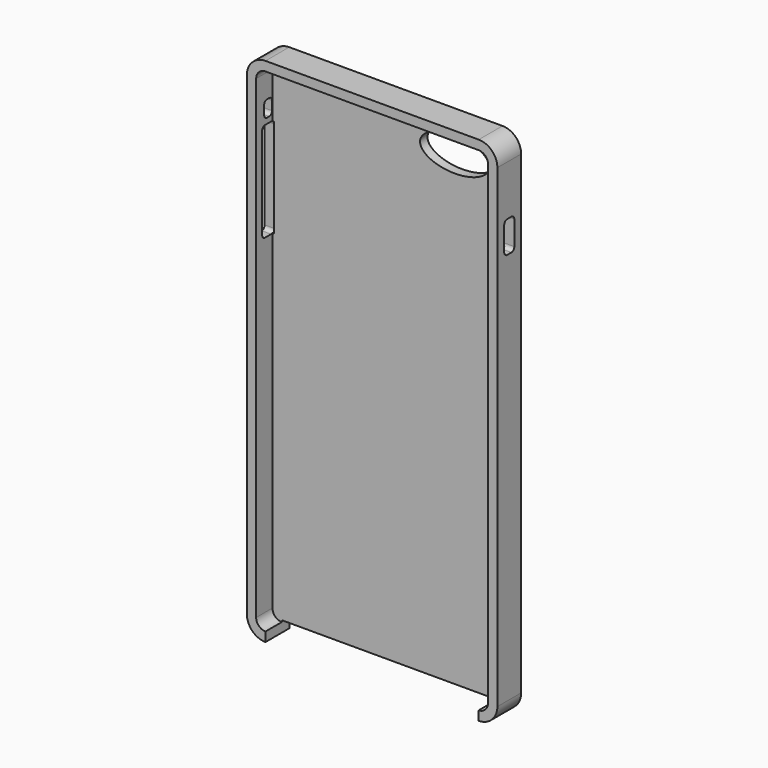
from build123d import *

# Parameters (mm, degrees)
F0_W          = 68.3
F0_H          = 139.5
F1_DEPTH      = 4.05
F2_R          = 5.08
F3_T          = -2.54
F5_DEPTH      = 30
F7_W          = 32.1311485022
F7_H          = 8.1
F8_DEPTH      = 3
F9_W          = 3.4326917958
F9_H          = 8.6012896579
F10_DEPTH     = 3
F11_W         = 2.6687926147
F11_H         = 4.4363630507
F12_DEPTH     = 3
F13_W         = 4.0359543636
F13_H         = 27.0408764482
F14_DEPTH     = 3
F15_W         = 16.4470494014
F15_H         = 8.1
F8_FACE_W     = 9.5618020964
F8_FACE_H     = 8.1
F16_DEPTH     = 3
F19_T1_DEPTH  = 2.54
F19_T3_DEPTH  = 2.54
F19_T8_DEPTH  = 3
F19_T14_DEPTH = 3
F19_T20_DEPTH = 3
F19_T26_DEPTH = 5.5
F19_T32_DEPTH = 3
F19_T38_DEPTH = 3
F19_T44_DEPTH = 3
F19_T50_DEPTH = 5.5
F19_T56_DEPTH = 5.5
F19_T62_DEPTH = 3
F19_T68_DEPTH = 3
F19_T74_DEPTH = 3
F19_T80_DEPTH = 5.5
F19_T86_DEPTH = 3
F19_T92_DEPTH = 3
F19_T98_DEPTH = 3


# Not quite as in the source:
# - a fillet or chamfer that OpenCascade refuses, or shapes differently, is made with other operations: its cross-section is extruded or revolved along the edge and cut away or added
# - a feature of the source that left no trace in its solid (it failed there, or was rolled back) is left out


with BuildPart() as f1:
    # F0 (on Front) → F1 (new body, symmetric)
    with BuildSketch(Plane.XZ):
        Rectangle(F0_W, F0_H)
    extrude(amount=F1_DEPTH, both=True)

    # F2
    f2_edges = [f1.edges().sort_by_distance(p)[0] for p in [
        (-34.15, 0, 69.75),
        (34.15, 0, 69.75),
        (34.15, 0, -69.75),
        (-34.15, 0, -69.75),
    ]]
    fillet(f2_edges, radius=F2_R)

    # F3
    f3_openings = [f1.faces().sort_by_distance(p)[0] for p in [
        (0, -4.05, 0),
    ]]
    offset(amount=F3_T, openings=f3_openings)

    # F4 (on face) → F5 (cut, symmetric)
    with BuildSketch(Plane.XZ.offset(-1.51)):
        with BuildLine():
            add(Edge.make_bspline(
                [(8.6272396147, 60.3893473744), (8.6272396147, 52.4417168684), (22.797036916, 56.4155321214), (36.9668342173, 60.3893473744), (22.797036916, 64.3631626275), (8.6272396147, 68.3369778805), (8.6272396147, 60.3893473744)],
                knots=[0, 0, 0, 2.0943951024, 2.0943951024, 4.1887902048, 4.1887902048, 6.2831853072, 6.2831853072, 6.2831853072], degree=2, weights=[1, 0.5, 1, 0.5, 1, 0.5, 1]))
        make_face()
    extrude(amount=F5_DEPTH, both=True, mode=Mode.SUBTRACT)

    # F7 (on face) → F8 (cut, symmetric)
    with BuildSketch(Plane(origin=(0, 0, -69.75), x_dir=(1, 0, 0), z_dir=(0, 0, -1))):
        with Locations((3.4426236525, 0)):
            Rectangle(F7_W, F7_H)
    extrude(amount=F8_DEPTH, both=True, mode=Mode.SUBTRACT)

    # F9 (on face) → F10 (cut, symmetric)
    with BuildSketch(Plane.YZ.offset(34.15)):
        with Locations((0, 46.6718673706)):
            Rectangle(F9_W, F9_H)
    extrude(amount=F10_DEPTH, both=True, mode=Mode.SUBTRACT)

    # F11 (on face) → F12 (cut, symmetric)
    with BuildSketch(Plane(origin=(-34.15, 0, 0), x_dir=(0, -1, 0), z_dir=(-1, 0, 0))):
        with Locations((0, 55.9940540446)):
            Rectangle(F11_W, F11_H)
    extrude(amount=F12_DEPTH, both=True, mode=Mode.SUBTRACT)

    # F13 (on face) → F14 (cut, symmetric)
    with BuildSketch(Plane(origin=(-34.15, 0, 0), x_dir=(0, -1, 0), z_dir=(-1, 0, 0))):
        with Locations((0, 38.7848801911)):
            Rectangle(F13_W, F13_H)
    extrude(amount=F14_DEPTH, both=True, mode=Mode.SUBTRACT)

    # F15 (on face) + F8_face (on face) → F16 (cut)
    with BuildSketch(Plane(origin=(0, 0, -69.75), x_dir=(1, 0, 0), z_dir=(0, 0, -1))):
        with Locations((-20.8464752993, 0)):
            Rectangle(F15_W, F15_H)
    with BuildSketch(Plane(origin=(-20.8464752993, 0, -69.75), x_dir=(1, 0, 0), z_dir=(0, 0, -1))):
        with Locations((45.1355742511, 0)):
            Rectangle(F8_FACE_W, F8_FACE_H)
    extrude(amount=-F16_DEPTH, mode=Mode.SUBTRACT)

    # F19: fillet of radius 1 on 12 edges, made by hand

    # F19_s2 → F19_t1 (join)
    with BuildSketch(Plane.YZ.offset(-34.15)):
        with BuildLine():
            ThreePointArc((0.3343963074, 58.21223557), (1.0415030885, 57.9193423511), (1.3343963074, 57.21223557))
            Line((1.3343963074, 57.21223557), (1.3343963074, 58.21223557))
            Line((1.3343963074, 58.21223557), (0.3343963074, 58.21223557))
        make_face()
        with BuildLine():
            ThreePointArc((1.3343963074, 54.7758725193), (1.0415030885, 54.0687657381), (0.3343963074, 53.7758725193))
            Line((0.3343963074, 53.7758725193), (1.3343963074, 53.7758725193))
            Line((1.3343963074, 53.7758725193), (1.3343963074, 54.7758725193))
        make_face()
        with BuildLine():
            ThreePointArc((-1.3343963074, 54.7758725193), (-1.0415030885, 54.0687657381), (-0.3343963074, 53.7758725193))
            Line((-0.3343963074, 53.7758725193), (-1.3343963074, 53.7758725193))
            Line((-1.3343963074, 53.7758725193), (-1.3343963074, 54.7758725193))
        make_face()
        with BuildLine():
            ThreePointArc((-0.3343963074, 58.21223557), (-1.0415030885, 57.9193423511), (-1.3343963074, 57.21223557))
            Line((-1.3343963074, 57.21223557), (-1.3343963074, 58.21223557))
            Line((-1.3343963074, 58.21223557), (-0.3343963074, 58.21223557))
        make_face()
        with BuildLine():
            ThreePointArc((-2.0179771818, 26.264441967), (-1.725083963, 25.5573351858), (-1.0179771818, 25.264441967))
            Line((-1.0179771818, 25.264441967), (-2.0179771818, 25.264441967))
            Line((-2.0179771818, 25.264441967), (-2.0179771818, 26.264441967))
        make_face()
        with BuildLine():
            ThreePointArc((-2.0179771818, 51.3053184152), (-1.725083963, 52.0124251964), (-1.0179771818, 52.3053184152))
            Line((-1.0179771818, 52.3053184152), (-2.0179771818, 52.3053184152))
            Line((-2.0179771818, 52.3053184152), (-2.0179771818, 51.3053184152))
        make_face()
    extrude(amount=F19_T1_DEPTH)

    # F19_s4 → F19_t3 (join)
    with BuildSketch(Plane.YZ.offset(31.61)):
        with BuildLine():
            ThreePointArc((-0.7163458979, 42.3712225417), (-1.4234526791, 42.6641157605), (-1.7163458979, 43.3712225417))
            Line((-1.7163458979, 43.3712225417), (-1.7163458979, 42.3712225417))
            Line((-1.7163458979, 42.3712225417), (-0.7163458979, 42.3712225417))
        make_face()
        with BuildLine():
            ThreePointArc((-1.7163458979, 49.9725121995), (-1.4234526791, 50.6796189807), (-0.7163458979, 50.9725121995))
            Line((-0.7163458979, 50.9725121995), (-1.7163458979, 50.9725121995))
            Line((-1.7163458979, 50.9725121995), (-1.7163458979, 49.9725121995))
        make_face()
    extrude(amount=F19_T3_DEPTH)


with BuildPart() as f19_tool6:
    # F19_s7 → F19_t8 (new body)
    with BuildSketch(Plane.YZ.offset(34.15)):
        with BuildLine():
            ThreePointArc((1.7163458979, 43.3712225417), (1.4234526791, 42.6641157605), (0.7163458979, 42.3712225417))
            Line((0.7163458979, 42.3712225417), (1.7163458979, 42.3712225417))
            Line((1.7163458979, 42.3712225417), (1.7163458979, 43.3712225417))
        make_face()
    extrude(amount=-F19_T8_DEPTH)

    split(bisect_by=Plane.XZ.offset(-1.51), keep=Keep.BOTTOM)

    split(bisect_by=Plane.YZ.offset(31.61), keep=Keep.TOP)


with BuildPart() as f1_1:
    add(f1.part)

    # F19_t5: union F19_tool6
    add(f19_tool6.part)


with BuildPart() as f19_tool12:
    # F19_s13 → F19_t14 (new body)
    with BuildSketch(Plane.YZ.offset(34.15)):
        with BuildLine():
            ThreePointArc((1.7163458979, 43.3712225417), (1.4234526791, 42.6641157605), (0.7163458979, 42.3712225417))
            Line((0.7163458979, 42.3712225417), (1.7163458979, 42.3712225417))
            Line((1.7163458979, 42.3712225417), (1.7163458979, 43.3712225417))
        make_face()
    extrude(amount=-F19_T14_DEPTH)

    split(bisect_by=Plane.XZ.offset(-1.51), keep=Keep.TOP)

    split(bisect_by=Plane.YZ.offset(31.61), keep=Keep.TOP)


with BuildPart() as f1_2:
    add(f1_1.part)

    # F19_t11: union F19_tool12
    add(f19_tool12.part)


with BuildPart() as f19_tool18:
    # F19_s19 → F19_t20 (new body)
    with BuildSketch(Plane.YZ.offset(34.15)):
        with BuildLine():
            ThreePointArc((1.7163458979, 43.3712225417), (1.4234526791, 42.6641157605), (0.7163458979, 42.3712225417))
            Line((0.7163458979, 42.3712225417), (1.7163458979, 42.3712225417))
            Line((1.7163458979, 42.3712225417), (1.7163458979, 43.3712225417))
        make_face()
    extrude(amount=-F19_T20_DEPTH)

    split(bisect_by=Plane.XZ.offset(-1.51), keep=Keep.BOTTOM)

    split(bisect_by=Plane.YZ.offset(31.61), keep=Keep.BOTTOM)


with BuildPart() as f1_3:
    add(f1_2.part)

    # F19_t17: union F19_tool18
    add(f19_tool18.part)


with BuildPart() as f19_tool24:
    # F19_s25 → F19_t26 (new body)
    with BuildSketch(Plane.YZ.offset(34.15)):
        with BuildLine():
            ThreePointArc((1.7163458979, 43.3712225417), (1.4234526791, 42.6641157605), (0.7163458979, 42.3712225417))
            Line((0.7163458979, 42.3712225417), (1.7163458979, 42.3712225417))
            Line((1.7163458979, 42.3712225417), (1.7163458979, 43.3712225417))
        make_face()
    extrude(amount=-F19_T26_DEPTH)

    split(bisect_by=Plane.YZ.offset(31.15), keep=Keep.BOTTOM)

    split(bisect_by=Plane.XZ.offset(-1.51), keep=Keep.BOTTOM)


with BuildPart() as f1_4:
    add(f1_3.part)

    # F19_t23: union F19_tool24
    add(f19_tool24.part)


with BuildPart() as f19_tool30:
    # F19_s31 → F19_t32 (new body)
    with BuildSketch(Plane.YZ.offset(34.15)):
        with BuildLine():
            ThreePointArc((1.7163458979, 49.9725121995), (1.4234526791, 50.6796189807), (0.7163458979, 50.9725121995))
            Line((0.7163458979, 50.9725121995), (1.7163458979, 50.9725121995))
            Line((1.7163458979, 50.9725121995), (1.7163458979, 49.9725121995))
        make_face()
    extrude(amount=-F19_T32_DEPTH)

    split(bisect_by=Plane.XZ.offset(-1.51), keep=Keep.BOTTOM)

    split(bisect_by=Plane.YZ.offset(31.61), keep=Keep.TOP)


with BuildPart() as f1_5:
    add(f1_4.part)

    # F19_t29: union F19_tool30
    add(f19_tool30.part)


with BuildPart() as f19_tool36:
    # F19_s37 → F19_t38 (new body)
    with BuildSketch(Plane.YZ.offset(34.15)):
        with BuildLine():
            ThreePointArc((1.7163458979, 49.9725121995), (1.4234526791, 50.6796189807), (0.7163458979, 50.9725121995))
            Line((0.7163458979, 50.9725121995), (1.7163458979, 50.9725121995))
            Line((1.7163458979, 50.9725121995), (1.7163458979, 49.9725121995))
        make_face()
    extrude(amount=-F19_T38_DEPTH)

    split(bisect_by=Plane.XZ.offset(-1.51), keep=Keep.TOP)

    split(bisect_by=Plane.YZ.offset(31.61), keep=Keep.TOP)


with BuildPart() as f1_6:
    add(f1_5.part)

    # F19_t35: union F19_tool36
    add(f19_tool36.part)


with BuildPart() as f19_tool42:
    # F19_s43 → F19_t44 (new body)
    with BuildSketch(Plane.YZ.offset(34.15)):
        with BuildLine():
            ThreePointArc((1.7163458979, 49.9725121995), (1.4234526791, 50.6796189807), (0.7163458979, 50.9725121995))
            Line((0.7163458979, 50.9725121995), (1.7163458979, 50.9725121995))
            Line((1.7163458979, 50.9725121995), (1.7163458979, 49.9725121995))
        make_face()
    extrude(amount=-F19_T44_DEPTH)

    split(bisect_by=Plane.XZ.offset(-1.51), keep=Keep.BOTTOM)

    split(bisect_by=Plane.YZ.offset(31.61), keep=Keep.BOTTOM)


with BuildPart() as f1_7:
    add(f1_6.part)

    # F19_t41: union F19_tool42
    add(f19_tool42.part)


with BuildPart() as f19_tool48:
    # F19_s49 → F19_t50 (new body)
    with BuildSketch(Plane.YZ.offset(34.15)):
        with BuildLine():
            ThreePointArc((1.7163458979, 49.9725121995), (1.4234526791, 50.6796189807), (0.7163458979, 50.9725121995))
            Line((0.7163458979, 50.9725121995), (1.7163458979, 50.9725121995))
            Line((1.7163458979, 50.9725121995), (1.7163458979, 49.9725121995))
        make_face()
    extrude(amount=-F19_T50_DEPTH)

    split(bisect_by=Plane.YZ.offset(31.15), keep=Keep.BOTTOM)

    split(bisect_by=Plane.XZ.offset(-1.51), keep=Keep.BOTTOM)


with BuildPart() as f1_8:
    add(f1_7.part)

    # F19_t47: union F19_tool48
    add(f19_tool48.part)


with BuildPart() as f19_tool54:
    # F19_s55 → F19_t56 (new body)
    with BuildSketch(Plane.YZ.offset(-28.65)):
        with BuildLine():
            ThreePointArc((2.0179771818, 51.3053184152), (1.725083963, 52.0124251964), (1.0179771818, 52.3053184152))
            Line((1.0179771818, 52.3053184152), (2.0179771818, 52.3053184152))
            Line((2.0179771818, 52.3053184152), (2.0179771818, 51.3053184152))
        make_face()
    extrude(amount=-F19_T56_DEPTH)

    split(bisect_by=Plane.XZ.offset(-1.51), keep=Keep.BOTTOM)

    split(bisect_by=Plane.YZ.offset(-31.15), keep=Keep.TOP)


with BuildPart() as f1_9:
    add(f1_8.part)

    # F19_t53: union F19_tool54
    add(f19_tool54.part)


with BuildPart() as f19_tool60:
    # F19_s61 → F19_t62 (new body)
    with BuildSketch(Plane.YZ.offset(-31.15)):
        with BuildLine():
            ThreePointArc((2.0179771818, 51.3053184152), (1.725083963, 52.0124251964), (1.0179771818, 52.3053184152))
            Line((1.0179771818, 52.3053184152), (2.0179771818, 52.3053184152))
            Line((2.0179771818, 52.3053184152), (2.0179771818, 51.3053184152))
        make_face()
    extrude(amount=-F19_T62_DEPTH)

    split(bisect_by=Plane.XZ.offset(-1.51), keep=Keep.BOTTOM)

    split(bisect_by=Plane.YZ.offset(-31.61), keep=Keep.TOP)


with BuildPart() as f1_10:
    add(f1_9.part)

    # F19_t59: union F19_tool60
    add(f19_tool60.part)


with BuildPart() as f19_tool66:
    # F19_s67 → F19_t68 (new body)
    with BuildSketch(Plane.YZ.offset(-31.15)):
        with BuildLine():
            ThreePointArc((2.0179771818, 51.3053184152), (1.725083963, 52.0124251964), (1.0179771818, 52.3053184152))
            Line((1.0179771818, 52.3053184152), (2.0179771818, 52.3053184152))
            Line((2.0179771818, 52.3053184152), (2.0179771818, 51.3053184152))
        make_face()
    extrude(amount=-F19_T68_DEPTH)

    split(bisect_by=Plane.XZ.offset(-1.51), keep=Keep.BOTTOM)

    split(bisect_by=Plane.YZ.offset(-31.61), keep=Keep.BOTTOM)


with BuildPart() as f1_11:
    add(f1_10.part)

    # F19_t65: union F19_tool66
    add(f19_tool66.part)


with BuildPart() as f19_tool72:
    # F19_s73 → F19_t74 (new body)
    with BuildSketch(Plane.YZ.offset(-31.15)):
        with BuildLine():
            ThreePointArc((2.0179771818, 51.3053184152), (1.725083963, 52.0124251964), (1.0179771818, 52.3053184152))
            Line((1.0179771818, 52.3053184152), (2.0179771818, 52.3053184152))
            Line((2.0179771818, 52.3053184152), (2.0179771818, 51.3053184152))
        make_face()
    extrude(amount=-F19_T74_DEPTH)

    split(bisect_by=Plane.XZ.offset(-1.51), keep=Keep.TOP)

    split(bisect_by=Plane.YZ.offset(-31.61), keep=Keep.BOTTOM)


with BuildPart() as f1_12:
    add(f1_11.part)

    # F19_t71: union F19_tool72
    add(f19_tool72.part)


with BuildPart() as f19_tool78:
    # F19_s79 → F19_t80 (new body)
    with BuildSketch(Plane.YZ.offset(-28.65)):
        with BuildLine():
            ThreePointArc((2.0179771818, 26.264441967), (1.725083963, 25.5573351858), (1.0179771818, 25.264441967))
            Line((1.0179771818, 25.264441967), (2.0179771818, 25.264441967))
            Line((2.0179771818, 25.264441967), (2.0179771818, 26.264441967))
        make_face()
    extrude(amount=-F19_T80_DEPTH)

    split(bisect_by=Plane.XZ.offset(-1.51), keep=Keep.BOTTOM)

    split(bisect_by=Plane.YZ.offset(-31.15), keep=Keep.TOP)


with BuildPart() as f1_13:
    add(f1_12.part)

    # F19_t77: union F19_tool78
    add(f19_tool78.part)


with BuildPart() as f19_tool84:
    # F19_s85 → F19_t86 (new body)
    with BuildSketch(Plane.YZ.offset(-31.15)):
        with BuildLine():
            ThreePointArc((2.0179771818, 26.264441967), (1.725083963, 25.5573351858), (1.0179771818, 25.264441967))
            Line((1.0179771818, 25.264441967), (2.0179771818, 25.264441967))
            Line((2.0179771818, 25.264441967), (2.0179771818, 26.264441967))
        make_face()
    extrude(amount=-F19_T86_DEPTH)

    split(bisect_by=Plane.XZ.offset(-1.51), keep=Keep.BOTTOM)

    split(bisect_by=Plane.YZ.offset(-31.61), keep=Keep.TOP)


with BuildPart() as f1_14:
    add(f1_13.part)

    # F19_t83: union F19_tool84
    add(f19_tool84.part)


with BuildPart() as f19_tool90:
    # F19_s91 → F19_t92 (new body)
    with BuildSketch(Plane.YZ.offset(-31.15)):
        with BuildLine():
            ThreePointArc((2.0179771818, 26.264441967), (1.725083963, 25.5573351858), (1.0179771818, 25.264441967))
            Line((1.0179771818, 25.264441967), (2.0179771818, 25.264441967))
            Line((2.0179771818, 25.264441967), (2.0179771818, 26.264441967))
        make_face()
    extrude(amount=-F19_T92_DEPTH)

    split(bisect_by=Plane.XZ.offset(-1.51), keep=Keep.BOTTOM)

    split(bisect_by=Plane.YZ.offset(-31.61), keep=Keep.BOTTOM)


with BuildPart() as f1_15:
    add(f1_14.part)

    # F19_t89: union F19_tool90
    add(f19_tool90.part)


with BuildPart() as f19_tool96:
    # F19_s97 → F19_t98 (new body)
    with BuildSketch(Plane.YZ.offset(-31.15)):
        with BuildLine():
            ThreePointArc((2.0179771818, 26.264441967), (1.725083963, 25.5573351858), (1.0179771818, 25.264441967))
            Line((1.0179771818, 25.264441967), (2.0179771818, 25.264441967))
            Line((2.0179771818, 25.264441967), (2.0179771818, 26.264441967))
        make_face()
    extrude(amount=-F19_T98_DEPTH)

    split(bisect_by=Plane.XZ.offset(-1.51), keep=Keep.TOP)

    split(bisect_by=Plane.YZ.offset(-31.61), keep=Keep.BOTTOM)


with BuildPart() as f1_16:
    add(f1_15.part)

    # F19_t95: union F19_tool96
    add(f19_tool96.part)


solid = f1_16.part
